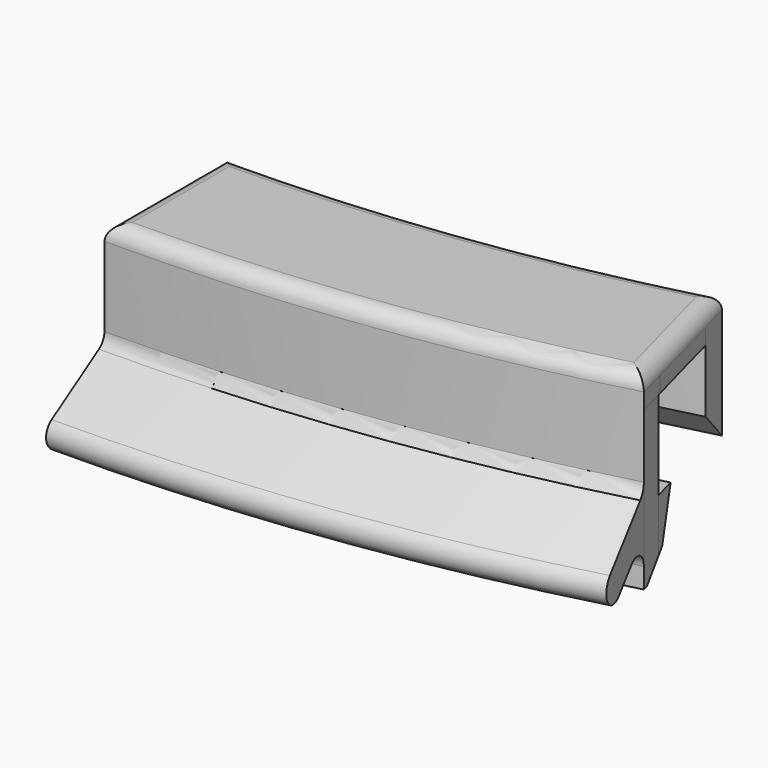
from build123d import *

# Parameters (mm, degrees)
F2_DEPTH      = 2.54
F3_DEPTH      = 7.62
F5_DEPTH      = 12.7
F7_ANGLE      = 15
F8_T2_ANGLE   = 20.2683164311
F8_T4_ANGLE   = 18.6436758241
F10_ANGLE     = 15
F11_T2_ANGLE  = 15
F11_T4_ANGLE  = 15
F11_T5_DEPTH  = 18.5785787418
F11_T7_DEPTH  = 18.5785787418
F11_T10_ANGLE = 17.3026091046
F11_T12_ANGLE = 17.3227523422
F11_T14_ANGLE = 17.3991627069
F11_T16_ANGLE = 17.6093282682


# Not quite as in the source:
# - a fillet or chamfer that OpenCascade refuses, or shapes differently, is made with other operations: its cross-section is extruded or revolved along the edge and cut away or added


with BuildPart() as f2:
    # F1 (on Top) → F2 (new body)
    with BuildSketch(Plane.XY):
        with BuildLine():
            ThreePointArc((36.1159330774, -134.7864972077), (18.2137880201, -138.3474552622), (0, -139.54125))
            Line((0, -139.54125), (0, -142.08125))
            ThreePointArc((0, -142.08125), (18.5453245484, -140.8657252101), (36.773333452, -137.2399488064))
            Line((36.773333452, -137.2399488064), (36.1159330774, -134.7864972077))
        make_face()
        with BuildLine():
            ThreePointArc((36.773333452, -137.2399488064), (18.5453245484, -140.8657252101), (0, -142.08125))
            Line((0, -142.08125), (0, -149.225))
            ThreePointArc((0, -149.225), (19.477771034, -147.9483594385), (38.6222720054, -144.140281428))
            Line((38.6222720054, -144.140281428), (36.773333452, -137.2399488064))
        make_face()
        with BuildLine():
            ThreePointArc((38.6222720054, -144.140281428), (19.477771034, -147.9483594385), (0, -149.225))
            Line((0, -149.225), (0, -151.765))
            ThreePointArc((0, -151.765), (19.8093075623, -150.4666293864), (39.27967238, -146.5937330268))
            Line((39.27967238, -146.5937330268), (38.6222720054, -144.140281428))
        make_face()
    extrude(amount=F2_DEPTH)

    # F1 (on Top) → F3 (join)
    with BuildSketch(Plane.XY):
        with BuildLine():
            ThreePointArc((36.1159330774, -134.7864972077), (18.2137880201, -138.3474552622), (0, -139.54125))
            Line((0, -139.54125), (0, -142.08125))
            ThreePointArc((0, -142.08125), (18.5453245484, -140.8657252101), (36.773333452, -137.2399488064))
            Line((36.773333452, -137.2399488064), (36.1159330774, -134.7864972077))
        make_face()
    extrude(amount=-F3_DEPTH)

    # F4 (on face) → F5 (join)
    with BuildSketch(Plane.XY):
        with BuildLine():
            ThreePointArc((38.6880120429, -144.3856265879), (19.5109246869, -148.2001864333), (0, -149.479))
            Line((0, -149.479), (0, -151.765))
            ThreePointArc((0, -151.765), (19.8093075623, -150.4666293864), (39.27967238, -146.5937330268))
            Line((39.27967238, -146.5937330268), (38.6880120429, -144.3856265879))
        make_face()
    extrude(amount=-F5_DEPTH)

    # F6 (on face) → F7 (revolve)
    with BuildSketch(Plane(origin=(0, 0, 0), x_dir=(0, -1, 0), z_dir=(-1, 0, 0))):
        Polygon((147.574, -7.112), (149.479, -12.7), (149.479, -7.112), align=None)
    revolve(axis=Axis((0, 0, 0), (0, 0, 1)), revolution_arc=F7_ANGLE)

    # F8: chamfer of 2.54 on 2 edges, made by hand

    # F8_s1 → F8_t2 (revolve, cut)
    with BuildSketch(Plane(origin=(0, 0, 0), x_dir=(0, 0, 1), z_dir=(-0.9989433481, 0.0459585396, 0))):
        Polygon((-7.62, -139.54125), (-5.08, -142.08125), (-7.62, -142.08125), align=None)
    revolve(axis=Axis((0, 0, -7.62), (0, 0, 1)), revolution_arc=F8_T2_ANGLE, mode=Mode.SUBTRACT)

    # F8_s3 → F8_t4 (revolve, cut)
    with BuildSketch(Plane(origin=(0, 0, 0), x_dir=(0, 0, 1), z_dir=(0.9572092654, 0.289396652, 0))):
        Polygon((-12.7, 151.2966330745), (-10.9795917766, 148.8924971966), (-12.7, 149.479), align=None)
    revolve(axis=Axis((0, 0, -12.7), (0, 0, -1)), revolution_arc=F8_T4_ANGLE, mode=Mode.SUBTRACT)

    # F9 (on face) → F10 (revolve)
    with BuildSketch(Plane(origin=(0, 0, 0), x_dir=(0, -1, 0), z_dir=(-1, 0, 0))):
        Polygon((158.1288493504, -9.8370487633), (151.765, -5.7552899175), (151.765, -8.7728602812), (156.7575335503, -11.9750602171), align=None)
        Polygon((151.765, -8.7728602812), (151.765, -5.7552899175), (151.765, 2.54), (139.54125, 2.54), (139.54125, -7.62), (142.08125, -5.08), (142.08125, 0), (149.479, 0), (149.479, -7.112), (147.574, -7.112), (148.8924971966, -10.9795917766), (151.2966330745, -12.7), (151.765, -12.7), align=None)
    revolve(axis=Axis((0, 0, 0), (0, 0, 1)), revolution_arc=F10_ANGLE)

    # F11: fillet of radius 1.27 on 8 edges, made by hand

    # F11_s1 → F11_t2 (revolve)
    with BuildSketch(Plane.YZ):
        with BuildLine():
            ThreePointArc((-151.7646, -5.0599866722), (-151.9205140931, -5.6702824854), (-152.3500463685, -6.1310125674))
            Line((-152.3500463685, -6.1310125674), (-152.2813510053, -6.2381151569))
            ThreePointArc((-152.2813510053, -6.2381151569), (-151.9889357987, -6.0500854846), (-151.6963046368, -5.862392507))
            Line((-151.6963046368, -5.862392507), (-151.63776, -5.7552899175))
            ThreePointArc((-151.63776, -5.7552899175), (-151.63776, -5.4076382949), (-151.63736, -5.0599866722))
            Line((-151.63736, -5.0599866722), (-151.7646, -5.0599866722))
        make_face()
    revolve(axis=Axis((0, 0, -5.7552899175), (0, 0, 1)), revolution_arc=F11_T2_ANGLE)

    # F11_s3 → F11_t4 (revolve)
    with BuildSketch(Plane.YZ):
        with BuildLine():
            ThreePointArc((-151.7646, -11.0968951513), (-152.4258553263, -9.9818406517), (-153.7214416132, -10.0272423808))
            Line((-153.7214416132, -10.0272423808), (-153.7900489045, -9.9202771037))
            ThreePointArc((-153.7900489045, -9.9202771037), (-152.8117201202, -9.2932544013), (-151.8336072912, -8.6658950041))
            Line((-151.8336072912, -8.6658950041), (-151.6379231299, -8.7728602812))
            ThreePointArc((-151.6379231299, -8.7728602812), (-151.6379231299, -9.9348777163), (-151.6375231299, -11.0968951513))
            Line((-151.6375231299, -11.0968951513), (-151.7646, -11.0968951513))
        make_face()
    revolve(axis=Axis((0, 0, -8.7728602812), (0, 0, 1)), revolution_arc=F11_T4_ANGLE)

    # F11_s6 → F11_t5 (cut)
    with BuildSketch(Plane.XZ.offset(136.3638356291)):
        with BuildLine():
            ThreePointArc((1.2709656854, 2.5404), (0.3719743879, 2.1680256121), (-0.0004, 1.2690343146))
            Line((-0.0004, 1.2690343146), (-0.1275365685, 1.2690343146))
            ThreePointArc((-0.1275365685, 1.2690343146), (-0.1271365685, 1.9045171573), (-0.1271365685, 2.54))
            Line((-0.1271365685, 2.54), (0, 2.6671365685))
            ThreePointArc((0, 2.6671365685), (0.6354828427, 2.6671365685), (1.2709656854, 2.6675365685))
            Line((1.2709656854, 2.6675365685), (1.2709656854, 2.5404))
        make_face()
    extrude(amount=F11_T5_DEPTH, mode=Mode.SUBTRACT)

    # F11_s8 → F11_t7 (cut)
    with BuildSketch(Plane(origin=(40.1020477334, -149.6628796285, 0), x_dir=(0, 0, 1), z_dir=(-0.2588190451, 0.9659258263, 0))):
        with BuildLine():
            ThreePointArc((1.2690343146, 0.0004), (2.1680256121, -0.3719743879), (2.5404, -1.2709656854))
            Line((2.5404, -1.2709656854), (2.6675365685, -1.2709656854))
            ThreePointArc((2.6675365685, -1.2709656854), (2.6671365685, -0.6354828427), (2.6671365685, 0))
            Line((2.6671365685, 0), (2.54, 0.1271365685))
            ThreePointArc((2.54, 0.1271365685), (1.9045171573, 0.1271365685), (1.2690343146, 0.1275365685))
            Line((1.2690343146, 0.1275365685), (1.2690343146, 0.0004))
        make_face()
    extrude(amount=F11_T7_DEPTH, mode=Mode.SUBTRACT)

    # F11_s9 → F11_t10 (revolve, cut)
    with BuildSketch(Plane(origin=(0, 0, 0), x_dir=(0, 0, 1), z_dir=(-0.9997981213, 0.0200927029, 0))):
        with BuildLine():
            ThreePointArc((-9.1505328065, -157.0592467258), (-9.9493287423, -157.6149202728), (-10.9070832984, -157.443006783))
            Line((-10.9070832984, -157.443006783), (-10.9757228201, -157.5500223104))
            ThreePointArc((-10.9757228201, -157.5500223104), (-10.440597575, -157.8927752468), (-9.9056882851, -158.2358648778))
            Line((-9.9056882851, -158.2358648778), (-9.7300332359, -158.1974888721))
            ThreePointArc((-9.7300332359, -158.1974888721), (-9.3869436048, -157.6625795822), (-9.043517279, -157.1278862476))
            Line((-9.043517279, -157.1278862476), (-9.1505328065, -157.0592467258))
        make_face()
    revolve(axis=Axis((0, 0, -9.8370487633), (0, 0, 1)), revolution_arc=F11_T10_ANGLE, mode=Mode.SUBTRACT)

    # F11_s11 → F11_t12 (revolve, cut)
    with BuildSketch(Plane(origin=(0, 0, 0), x_dir=(0, 0, 1), z_dir=(-0.9997945739, 0.02026845, 0))):
        with BuildLine():
            ThreePointArc((-10.9054575925, -157.4440495071), (-11.4611311395, -156.6452535713), (-11.2892176497, -155.6874990152))
            Line((-11.2892176497, -155.6874990152), (-11.3962331771, -155.6188594935))
            ThreePointArc((-11.3962331771, -155.6188594935), (-11.7389861135, -156.1539847386), (-12.0820757445, -156.6888940285))
            Line((-12.0820757445, -156.6888940285), (-12.0436997388, -156.8645490777))
            ThreePointArc((-12.0436997388, -156.8645490777), (-11.5087904489, -157.2076387088), (-10.9740971142, -157.5510650346))
            Line((-10.9740971142, -157.5510650346), (-10.9054575925, -157.4440495071))
        make_face()
    revolve(axis=Axis((0, 0, -11.9750602171), (0, 0, 1)), revolution_arc=F11_T12_ANGLE, mode=Mode.SUBTRACT)

    # F11_s13 → F11_t14 (revolve, cut)
    with BuildSketch(Plane(origin=(0, 0, 0), x_dir=(0, 0, 1), z_dir=(-0.9997808365, 0.0209351147, 0))):
        with BuildLine():
            ThreePointArc((2.5404, -150.4940343146), (2.1680256121, -151.3930256121), (1.2690343146, -151.7654))
            Line((1.2690343146, -151.7654), (1.2690343146, -151.8925365685))
            ThreePointArc((1.2690343146, -151.8925365685), (1.9045171573, -151.8921365685), (2.54, -151.8921365685))
            Line((2.54, -151.8921365685), (2.6671365685, -151.765))
            ThreePointArc((2.6671365685, -151.765), (2.6671365685, -151.1295171573), (2.6675365685, -150.4940343146))
            Line((2.6675365685, -150.4940343146), (2.5404, -150.4940343146))
        make_face()
    revolve(axis=Axis((0, 0, 2.54), (0, 0, 1)), revolution_arc=F11_T14_ANGLE, mode=Mode.SUBTRACT)

    # F11_s15 → F11_t16 (revolve, cut)
    with BuildSketch(Plane(origin=(0, 0, 0), x_dir=(0, 0, 1), z_dir=(0.9597824413, 0.2807448405, 0))):
        with BuildLine():
            ThreePointArc((1.2690343146, 139.54085), (2.1680256121, 139.9132243879), (2.5404, 140.8122156854))
            Line((2.5404, 140.8122156854), (2.6675365685, 140.8122156854))
            ThreePointArc((2.6675365685, 140.8122156854), (2.6671365685, 140.1767328427), (2.6671365685, 139.54125))
            Line((2.6671365685, 139.54125), (2.54, 139.4141134315))
            ThreePointArc((2.54, 139.4141134315), (1.9045171573, 139.4141134315), (1.2690343146, 139.4137134315))
            Line((1.2690343146, 139.4137134315), (1.2690343146, 139.54085))
        make_face()
    revolve(axis=Axis((0, 0, 2.54), (0, 0, -1)), revolution_arc=F11_T16_ANGLE, mode=Mode.SUBTRACT)


solid = f2.part
